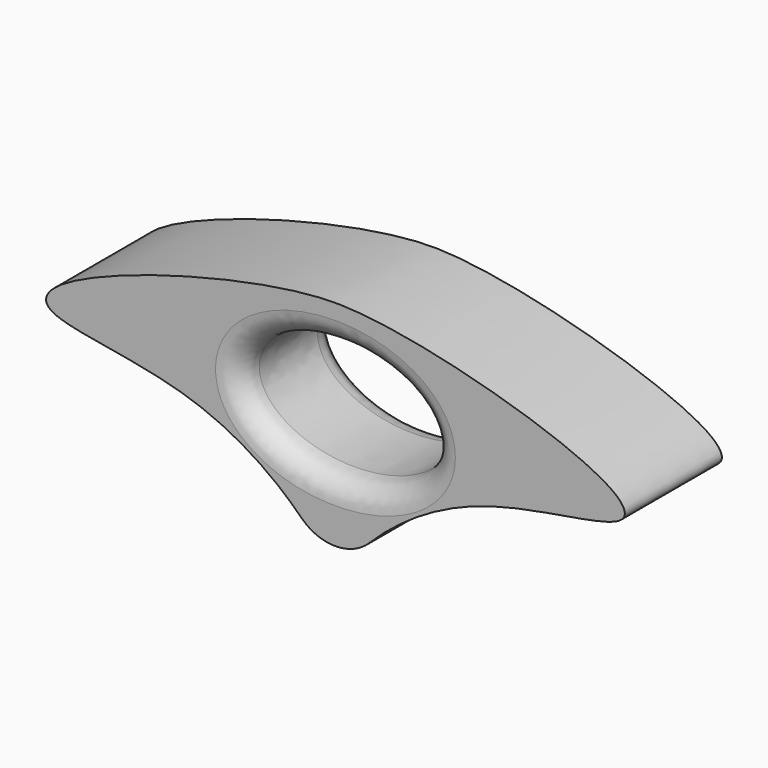
from build123d import *

# Parameters (mm, degrees)
F2_DEPTH = 12.7
F3_R     = 5.08
F4_R     = 2.54


with BuildPart() as f2:
    # F1 (on face) → F2 (new body)
    with BuildSketch(Plane.XZ):
        with BuildLine():
            add(Edge.make_bspline(
                [(0, -15.3768792944), (-2.6452205572, -10.7952228921), (-12.982730275, -1.7308159859), (-31.7412708843, -1.4312284761), (-28.6135466039, 4.4016031246), (-7.9863189249, 10.16), (0, 10.16)],
                knots=[0, 0, 0, 0, 0.2820658497, 0.5371636389, 0.6475302664, 1, 1, 1, 1], degree=3))
            add(Edge.make_bspline(
                [(0, -15.3768792944), (2.6452205572, -10.7952228921), (12.982730275, -1.7308159859), (31.7412708843, -1.4312284761), (28.6135466039, 4.4016031246), (7.9863189249, 10.16), (0, 10.16)],
                knots=[0, 0, 0, 0, 0.2820658497, 0.5371636389, 0.6475302664, 1, 1, 1, 1], degree=3))
        make_face()
        with BuildLine():
            add(Edge.make_bspline(
                [(10, 0), (10, 10.3923048454), (-5, 5.1961524227), (-20, 0), (-5, -5.1961524227), (10, -10.3923048454), (10, 0)],
                knots=[0, 0, 0, 2.0943951024, 2.0943951024, 4.1887902048, 4.1887902048, 6.2831853072, 6.2831853072, 6.2831853072], degree=2, weights=[1, 0.5, 1, 0.5, 1, 0.5, 1]))
        make_face(mode=Mode.SUBTRACT)
    extrude(amount=F2_DEPTH)

    # F3
    f3_edges = [f2.edges().sort_by_distance(p)[0] for p in [
        (0, -6.35, -15.376879),
    ]]
    fillet(f3_edges, radius=F3_R)

    # F4
    f4_edges = [f2.edges().sort_by_distance(p)[0] for p in [
        (-10, -12.7, 0),
        (-10, 0, 0),
    ]]
    fillet(f4_edges, radius=F4_R)


solid = f2.part
